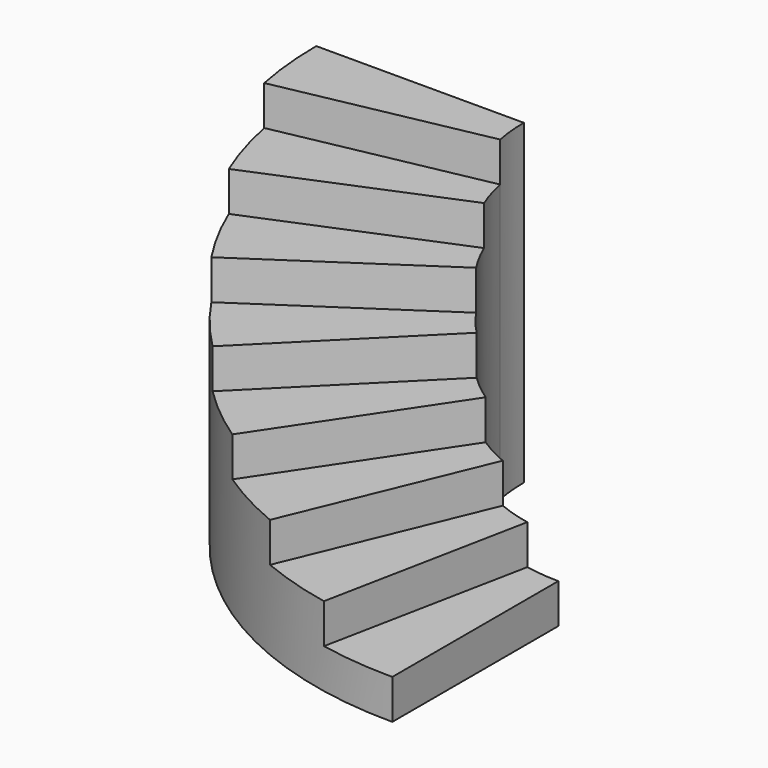
from build123d import *

# Parameters (mm, degrees)
F10_DEPTH = 254
F11_DEPTH = 508
F12_DEPTH = 762
F13_DEPTH = 1016
F14_DEPTH = 1270
F15_DEPTH = 1524
F16_DEPTH = 1778
F17_DEPTH = 2032


# Not quite as in the source:
# - a variable given as a bare number and used for a length is read in inches; the dataset says mm whatever the document's units were


with BuildPart() as f10:
    # F2 (on Top) → F10 (new body)
    with BuildSketch(Plane.XY):
        with BuildLine():
            Line((-979.52713178, -1331.3833333333), (-979.52713178, 0))
            ThreePointArc((-979.52713178, 0), (-1088.0337397438, 5.3305878284), (-1195.4953697572, 21.271014839))
            Line((-1195.4953697572, 21.271014839), (-1455.2353729841, -1284.5301610686))
            ThreePointArc((-1455.2353729841, -1284.5301610686), (-1218.5321267596, -1319.6417708508), (-979.52713178, -1331.3833333333))
        make_face()
    extrude(amount=F10_DEPTH)

    # F3 (on Top) → F11 (join)
    with BuildSketch(Plane.XY):
        with BuildLine():
            Line((-1455.2353729841, -1284.5301610686), (-1195.4953697572, 21.271014839))
            ThreePointArc((-1195.4953697572, 21.271014839), (-1300.8771075786, 47.6677660055), (-1403.1640694653, 84.2666261845))
            Line((-1403.1640694653, 84.2666261845), (-1912.662413259, -1145.7711854089))
            ThreePointArc((-1912.662413259, -1145.7711854089), (-1687.3572887973, -1226.3866479828), (-1455.2353729841, -1284.5301610686))
        make_face()
    extrude(amount=F11_DEPTH)

    # F4 (on Top) → F12 (join)
    with BuildSketch(Plane.XY):
        with BuildLine():
            Line((-1912.662413259, -1145.7711854089), (-1403.1640694653, 84.2666261845))
            ThreePointArc((-1403.1640694653, 84.2666261845), (-1501.3711760586, 130.7151283453), (-1594.5526392366, 186.5659480209))
            Line((-1594.5526392366, 186.5659480209), (-2334.229587975, -920.4388359719))
            ThreePointArc((-2334.229587975, -920.4388359719), (-2128.9809348565, -1043.4601443204), (-1912.662413259, -1145.7711854089))
        make_face()
    extrude(amount=F12_DEPTH)

    # F5 (on Top) → F13 (join)
    with BuildSketch(Plane.XY):
        with BuildLine():
            Line((-2334.229587975, -920.4388359719), (-1594.5526392366, 186.5659480209))
            ThreePointArc((-1594.5526392366, 186.5659480209), (-1681.8110705705, 251.2812112866), (-1762.3061236665, 324.2376747801))
            Line((-1762.3061236665, 324.2376747801), (-2703.7363070253, -617.1925085786))
            ThreePointArc((-2703.7363070253, -617.1925085786), (-2526.4317158846, -777.892022813), (-2334.229587975, -920.4388359719))
        make_face()
    extrude(amount=F13_DEPTH)

    # F6 (on Top) → F14 (join)
    with BuildSketch(Plane.XY):
        with BuildLine():
            Line((-2703.7363070253, -617.1925085786), (-1762.3061236665, 324.2376747801))
            ThreePointArc((-1762.3061236665, 324.2376747801), (-1835.2625871601, 404.7327278761), (-1899.9778504258, 491.9911592101))
            Line((-1899.9778504258, 491.9911592101), (-3006.9826344185, -247.6857895283))
            ThreePointArc((-3006.9826344185, -247.6857895283), (-2864.4358212597, -439.887917438), (-2703.7363070253, -617.1925085786))
        make_face()
    extrude(amount=F14_DEPTH)

    # F7 (on Top) → F15 (join)
    with BuildSketch(Plane.XY):
        with BuildLine():
            Line((-3006.9826344185, -247.6857895283), (-1899.9778504258, 491.9911592101))
            ThreePointArc((-1899.9778504258, 491.9911592101), (-1955.8286701014, 585.172622388), (-2002.2771722622, 683.3797289813))
            Line((-2002.2771722622, 683.3797289813), (-3232.3149838555, 173.8813851876))
            ThreePointArc((-3232.3149838555, 173.8813851876), (-3130.003942767, -42.4371364098), (-3006.9826344185, -247.6857895283))
        make_face()
    extrude(amount=F15_DEPTH)

    # F8 (on Top) → F16 (join)
    with BuildSketch(Plane.XY):
        with BuildLine():
            Line((-3232.3149838555, 173.8813851876), (-2002.2771722622, 683.3797289813))
            ThreePointArc((-2002.2771722622, 683.3797289813), (-2038.8760324411, 785.666690868), (-2065.2727836077, 891.0484286894))
            Line((-2065.2727836077, 891.0484286894), (-3371.0739595152, 631.3084254625))
            ThreePointArc((-3371.0739595152, 631.3084254625), (-3312.9304464294, 399.1865096494), (-3232.3149838555, 173.8813851876))
        make_face()
    extrude(amount=F16_DEPTH)

    # F9 (on Top) → F17 (join)
    with BuildSketch(Plane.XY):
        with BuildLine():
            Line((-3371.0739595152, 631.3084254625), (-2065.2727836077, 891.0484286894))
            ThreePointArc((-2065.2727836077, 891.0484286894), (-2081.2132106182, 998.5100587028), (-2086.5437984467, 1107.0166666667))
            Line((-2086.5437984467, 1107.0166666667), (-3417.92713178, 1107.0166666667))
            ThreePointArc((-3417.92713178, 1107.0166666667), (-3406.1855692975, 868.0116716871), (-3371.0739595152, 631.3084254625))
        make_face()
    extrude(amount=F17_DEPTH)


solid = f10.part
